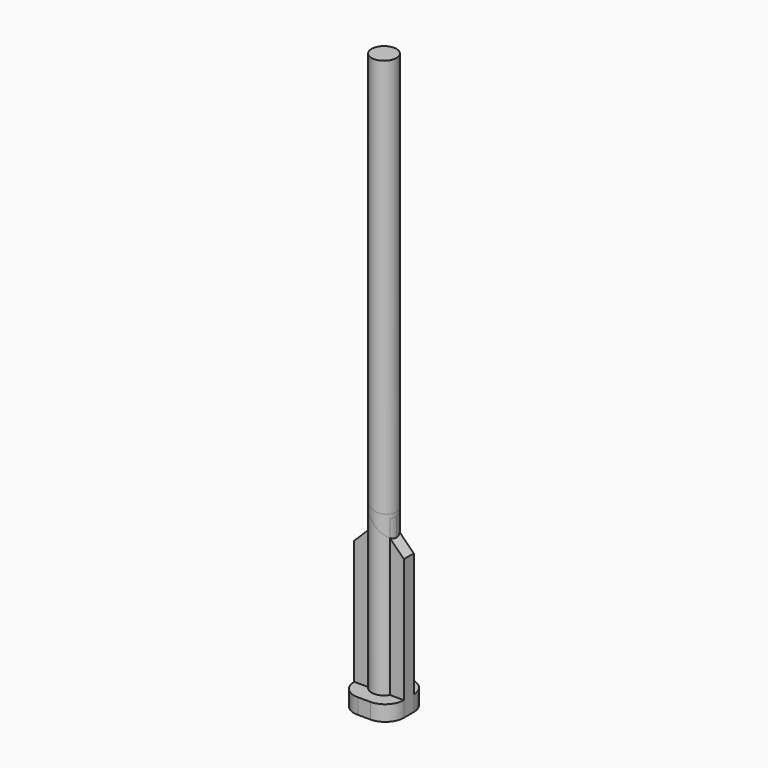
from build123d import *

# Parameters (mm, degrees)
F0_W         = 8
F0_H         = 8
F1_DEPTH     = 2.5
F2_R         = 3
F3_R         = 2
F4_DEPTH     = 90
F5_W         = 8
F5_H         = 2
F6_DEPTH     = 25
F7_T4_DEPTH  = 32.7638593636
F7_S5_R      = 2
F7_T6_DEPTH  = 19
F7_T10_DEPTH = 32.7638593636
F7_S11_R     = 2
F7_T12_DEPTH = 19


# Not quite as in the source:
# - a fillet or chamfer that OpenCascade refuses, or shapes differently, is made with other operations: its cross-section is extruded or revolved along the edge and cut away or added


with BuildPart() as f1:
    # F0 (on Top) → F1 (new body)
    with BuildSketch(Plane.XY):
        with Locations((-11.3665966003, 7.8844996169)):
            Rectangle(F0_W, F0_H)
    extrude(amount=F1_DEPTH)

    # F2
    f2_edges = [f1.edges().sort_by_distance(p)[0] for p in [
        (-15.366597, 3.8845, 1.25),
        (-15.366597, 11.8845, 1.25),
        (-7.366597, 3.8845, 1.25),
        (-7.366597, 11.8845, 1.25),
    ]]
    fillet(f2_edges, radius=F2_R)

    # F3 (on face) → F4 (join)
    with BuildSketch(Plane.XY.offset(2.5)):
        with Locations((-11.3665966003, 7.8844996169)):
            Circle(F3_R)
    extrude(amount=F4_DEPTH)

    # F5 (on face) → F6 (join)
    with BuildSketch(Plane.XY.offset(2.5)):
        with Locations((-11.3665966003, 7.8844996169)):
            Rectangle(F5_W, F5_H)
    extrude(amount=F6_DEPTH)

    # F7: chamfer of 5 on 2 edges, made by hand


with BuildPart() as f7_tool2:
    # F7_s3 → F7_t4 (new body)
    with BuildSketch(Plane.XZ.offset(-24.2664292987)):
        with BuildLine():
            Line((-16.427256772, 21.4393398282), (-9.3059364285, 28.5606601718))
            Line((-9.3059364285, 28.5606601718), (-9.3059364285, 29.3106601718))
            ThreePointArc((-9.3059364285, 29.3106601718), (-12.3362665144, 28.25), (-15.3665966003, 28.25))
            Line((-15.3665966003, 28.25), (-16.1165966003, 27.5))
            ThreePointArc((-16.1165966003, 27.5), (-16.1165966003, 24.4696699141), (-17.177256772, 21.4393398282))
            Line((-17.177256772, 21.4393398282), (-16.427256772, 21.4393398282))
        make_face()
    extrude(amount=F7_T4_DEPTH)

    # F7_s5 → F7_t6 (cut, symmetric)
    with BuildSketch(Plane.XY.offset(25.4)):
        with Locations((-11.3665966003, 7.8844996169)):
            Circle(F7_S5_R)
    extrude(amount=F7_T6_DEPTH, both=True, mode=Mode.SUBTRACT)


with BuildPart() as f1_1:
    add(f1.part)

    # F7_t1: cut F7_tool2
    add(f7_tool2.part, mode=Mode.SUBTRACT)


with BuildPart() as f7_tool8:
    # F7_s9 → F7_t10 (new body)
    with BuildSketch(Plane.XZ.offset(8.4974300649)):
        with BuildLine():
            Line((-6.3059364285, 21.4393398282), (-13.427256772, 28.5606601718))
            Line((-13.427256772, 28.5606601718), (-13.427256772, 29.3106601718))
            ThreePointArc((-13.427256772, 29.3106601718), (-10.3969266861, 28.25), (-7.3665966003, 28.25))
            Line((-7.3665966003, 28.25), (-6.6165966003, 27.5))
            ThreePointArc((-6.6165966003, 27.5), (-6.6165966003, 24.4696699141), (-5.5559364285, 21.4393398282))
            Line((-5.5559364285, 21.4393398282), (-6.3059364285, 21.4393398282))
        make_face()
    extrude(amount=-F7_T10_DEPTH)

    # F7_s11 → F7_t12 (cut, symmetric)
    with BuildSketch(Plane.XY.offset(25.4)):
        with Locations((-11.3665966003, 7.8844996169)):
            Circle(F7_S11_R)
    extrude(amount=F7_T12_DEPTH, both=True, mode=Mode.SUBTRACT)


with BuildPart() as f1_2:
    add(f1_1.part)

    # F7_t7: cut F7_tool8
    add(f7_tool8.part, mode=Mode.SUBTRACT)


solid = f1_2.part
